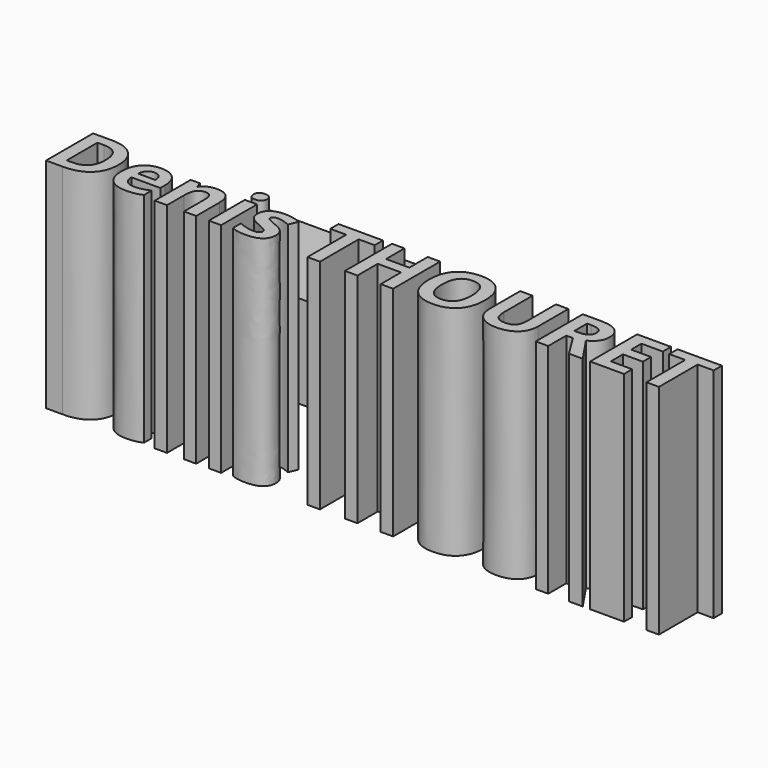
from build123d import *

# Parameters (mm, degrees)
F0_W         = 49.1070635617
F0_H         = 27.9486197978
F1_DEPTH     = 25.4
F4_TEXT_SIZE = 22.5368214564
F5_DEPTH     = 59.69


# Not quite as in the source:
# - the program builds the solid bodies; features that only make, move or delete a surface that nothing else refers to are left out
# - Text() gives the source's letters only with a copy of the font that has no kerning and outlines rounded to 1/6400 em; it was checked with that copy


with BuildPart() as f1:
    # F0 (on Top) → F1 (new body)
    with BuildSketch(Plane.XY):
        with Locations((-4.9788299948, 13.9743098989)):
            Rectangle(F0_W, F0_H)
    extrude(amount=F1_DEPTH)


with BuildPart() as f5:
    # F4 (on Top) → F5 (new body)
    with BuildSketch(Plane.XY):
        with Locations((-37.9901751876, -35.3929698467)):
            Text('Denis THOURET', F4_TEXT_SIZE, font='Open Sans', font_style=FontStyle.BOLD, text_align=(TextAlign.LEFT, TextAlign.BOTTOM))
    extrude(amount=F5_DEPTH)


solid = Compound([f1.part, f5.part])
